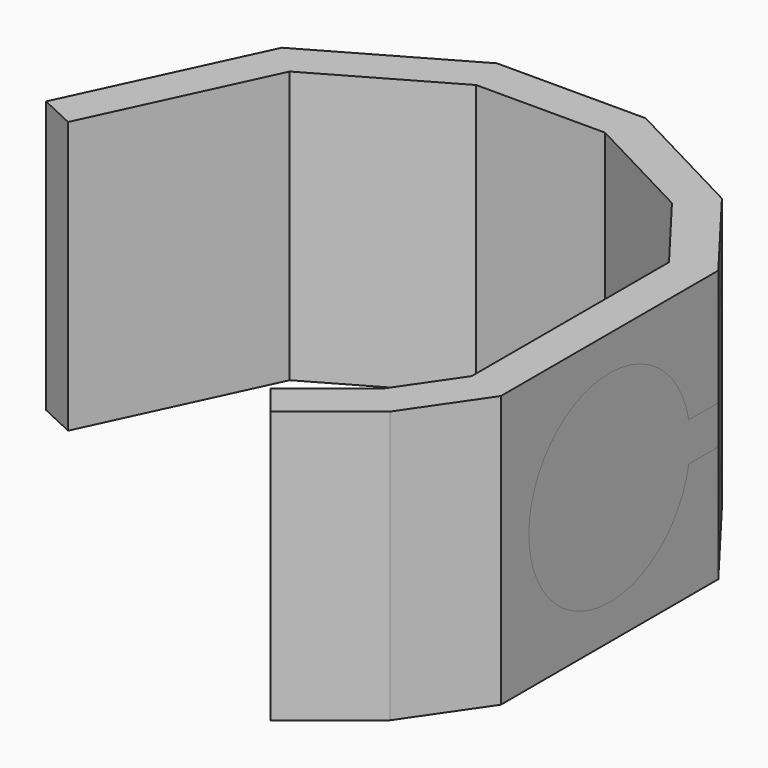
from build123d import *

# Parameters (mm, degrees)
F1_DEPTH = 35
F4_DEPTH = 4
F6_DEPTH = 91.8859431967


with BuildPart() as f1:
    # F0 (on Top) → F1 (new body)
    with BuildSketch(Plane.XY):
        Polygon((0, -35), (0, 0), (-9.5109246434, 12.4721351717), (-26.4208839566, 21.3360726107), (-45.5791160434, 21.3360726107), (-64.5962424722, 10.468820434), (-75.7963384867, -13.4686921408), (-71.2675436887, -15.5876648791), (-60.7392186918, 6.9140986486), (-44.2512588756, 16.336069832), (-27.6519096337, 16.336069832), (-12.8143973034, 8.5584768402), (-5.0000027788, -1.6889163893), (-5.0000027788, -33.4502943559), (-10.2991251018, -41.1776865134), (-19.1134621113, -48.2309964282), (-15.9894881577, -52.1349450095), (-6.5954562437, -44.617758139), align=None)
    extrude(amount=F1_DEPTH)


with BuildPart() as f2_1:
    # F2: copy of F1
    add(f1.part)

    # F3 (on face) → F4 (cut)
    with BuildSketch(Plane.YZ):
        with BuildLine():
            Line((0, 20), (-4.7426491778, 20))
            ThreePointArc((-4.7426491778, 20), (-30.5, 17.5), (-4.7426491778, 15))
            Line((-4.7426491778, 15), (0, 15))
            Line((0, 15), (0, 20))
        make_face()
    extrude(amount=-F4_DEPTH, mode=Mode.SUBTRACT)

    # F5 (on face) → F6 (cut, through all)
    with BuildSketch(Plane(origin=(0, 0, 0), x_dir=(-0.6063798108, 0.7951751537, 0), z_dir=(0.7951751537, 0.6063798108, 0))):
        Polygon((0, 20), (0, 17.5), (0, 15), (0, 7.5), (15.6847646879, 7.5), (15.6847646879, 27.5), (0, 27.5), align=None)
    extrude(amount=-F6_DEPTH, mode=Mode.SUBTRACT)


solid = Compound([f1.part, f2_1.part])
